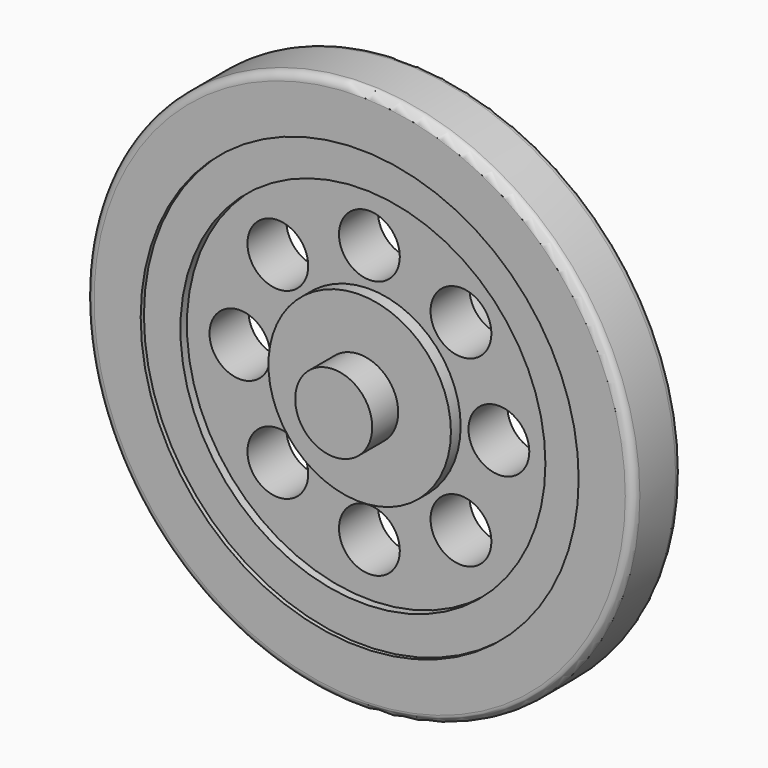
from build123d import *

# Parameters (mm, degrees)
F0_R      = 17.145
F1_DEPTH  = 3.81
F2_R      = 13.716
F2_R_2    = 11.43
F3_DEPTH  = 0.254
F4_DEPTH  = 0.762
F5_R      = 5.715
F6_DEPTH  = 0.762
F8_R      = 1.905
F9_DEPTH  = 25.4
F10_R     = 2.413
F11_DEPTH = 2.032
F14_R     = 3.175
F15_DEPTH = 8.89
F16_R     = 1.905
F17_DEPTH = 8.89
F18_R     = 0.508
F19_R     = 0.508


# Not quite as in the source:
# - the program builds the solid bodies; features that only make, move or delete a surface that nothing else refers to are left out


with BuildPart() as f1:
    # F0 (on Front) → F1 (new body)
    with BuildSketch(Plane.XZ):
        Circle(F0_R)
    extrude(amount=F1_DEPTH)

    # F2 (on face) → F3 (cut)
    with BuildSketch(Plane.XZ.offset(3.81)):
        Circle(F2_R)
        Circle(F2_R_2, mode=Mode.SUBTRACT)
    extrude(amount=-F3_DEPTH, mode=Mode.SUBTRACT)

    # F4 (cut): a face of the model
    f4_faces = [f1.faces().sort_by_distance(p)[0] for p in [
        (0, -3.81, 0),
    ]]
    extrude(f4_faces, amount=-F4_DEPTH, mode=Mode.SUBTRACT)

    # F5 (on face) → F6 (join)
    with BuildSketch(Plane.XZ.offset(3.048)):
        Circle(F5_R)
    extrude(amount=F6_DEPTH)

    # F8 (on face) → F9 (cut)
    with BuildSketch(Plane.XZ.offset(3.048)):
        with Locations((0, 8.1100180022)):
            Circle(F8_R)
        with Locations((-5.7346487249, 5.7346487249)):
            Circle(F8_R)
        with Locations((-5.7346487249, -5.7346487249)):
            Circle(F8_R)
        with Locations((0, -8.1100180022)):
            Circle(F8_R)
        with Locations((5.7346487249, -5.7346487249)):
            Circle(F8_R)
        with Locations((8.1100180022, 0)):
            Circle(F8_R)
        with Locations((5.7346487249, 5.7346487249)):
            Circle(F8_R)
        with Locations((-8.1100180022, 0)):
            Circle(F8_R)
    extrude(amount=-F9_DEPTH, mode=Mode.SUBTRACT)

    # F10 (on face) → F11 (join)
    with BuildSketch(Plane.XZ.offset(3.81)):
        Circle(F10_R)
    extrude(amount=F11_DEPTH)

    # F14 (on Front) → F15 (join)
    with BuildSketch(Plane.XZ):
        Circle(F14_R)
    extrude(amount=-F15_DEPTH)

    # F16 (on face) → F17 (cut)
    with BuildSketch(Plane(origin=(0, 8.89, 0), x_dir=(-1, 0, 0), z_dir=(0, 1, 0))):
        Circle(F16_R)
    extrude(amount=-F17_DEPTH, mode=Mode.SUBTRACT)

    # F18
    f18_edges = [f1.edges().sort_by_distance(p)[0] for p in [
        (-17.145, -3.81, 0),
    ]]
    fillet(f18_edges, radius=F18_R)

    # F19
    f19_edges = [f1.edges().sort_by_distance(p)[0] for p in [
        (-17.145, 0, 0),
    ]]
    fillet(f19_edges, radius=F19_R)


solid = f1.part
